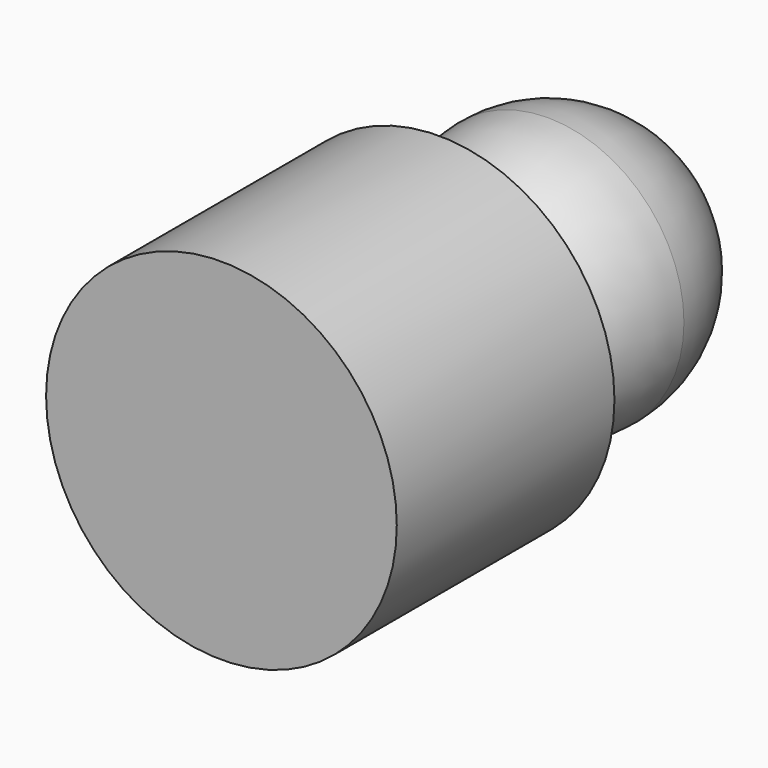
from build123d import *

# Parameters (mm, degrees)
F0_R     = 12.7
F1_DEPTH = 12.7
F2_R     = 12.69999
F4_R     = 16.3703
F5_DEPTH = 25.4


# Not quite as in the source:
# - a fillet or chamfer is up to 0.001 mm smaller than in the source, because OpenCascade refuses the exact size


with BuildPart() as f1:
    # F0 (on Front) → F1 (new body, symmetric)
    with BuildSketch(Plane.XZ):
        Circle(F0_R)
    extrude(amount=F1_DEPTH, both=True)

    # F2 (radius 12.7 in the source; OpenCascade refuses exactly that, so slightly less here)
    f2_edges = [f1.edges().sort_by_distance(p)[0] for p in [
        (-12.7, -12.7, 0),
        (-12.7, 12.7, 0),
    ]]
    fillet(f2_edges, radius=F2_R)


with BuildPart() as f5:
    # F4 (on offset) → F5 (new body)
    with BuildSketch(Plane.XZ.offset(12.7)):
        Circle(F4_R)
    extrude(amount=F5_DEPTH)


solid = Compound([f1.part, f5.part])
